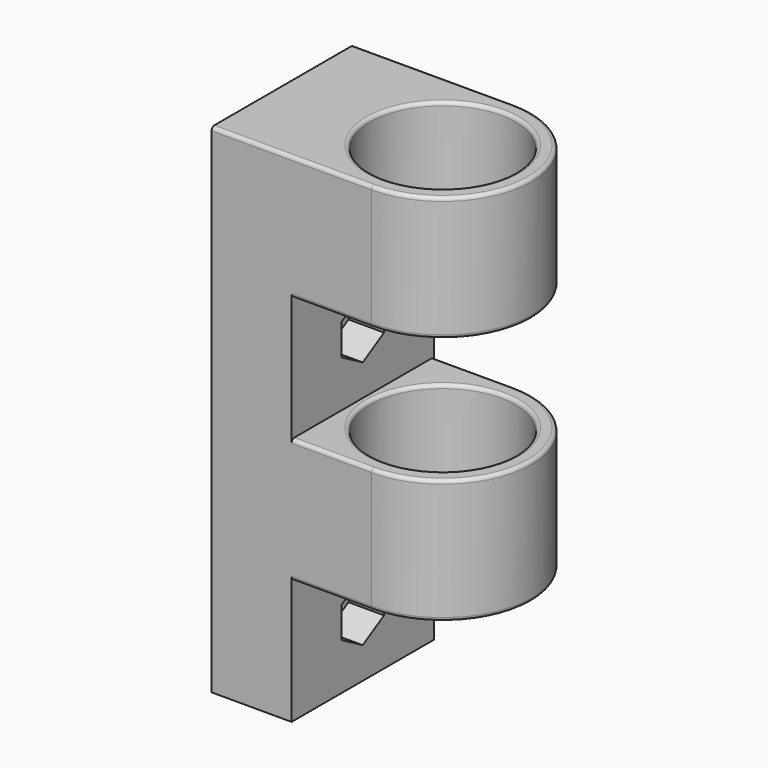
from build123d import *

# Parameters (mm, degrees)
F0_R     = 10.25
F1_DEPTH = 70
F2_W     = 11.25
F2_H     = 17.5
F2_W_2   = 18.7990599871
F3_DEPTH = 30
F4_R     = 2.1
F5_DEPTH = 5
F6_DEPTH = 11.251
F7_R     = 2.1
F8_DEPTH = 5
F9_DEPTH = 11.251
F10_R    = 0.5


# Not quite as in the source:
# - a feature names something its author has since deleted; it is built from what else it names


with BuildPart() as f1:
    # F0 (on Top) → F1 (new body)
    with BuildSketch(Plane.XY):
        with BuildLine():
            Line((0, 25), (0, 0))
            Line((0, 0), (22.5, 0))
            ThreePointArc((22.5, 0), (35, 12.5), (22.5, 25))
            Line((22.5, 25), (0, 25))
        make_face()
        with Locations((22.5, 12.5)):
            Circle(F0_R, mode=Mode.SUBTRACT)
    extrude(amount=F1_DEPTH)

    # F2 (on face) → F3 (cut)
    with BuildSketch(Plane.XZ):
        with Locations((16.875, 8.75)):
            Rectangle(F2_W, F2_H)
        with Locations((31.8995299935, 8.75)):
            Rectangle(F2_W_2, F2_H)
        with Locations((16.875, 43.75)):
            Rectangle(F2_W, F2_H)
        with Locations((31.8995299935, 43.75)):
            Rectangle(F2_W_2, F2_H)
    extrude(amount=-F3_DEPTH, mode=Mode.SUBTRACT)

    # F4 (on face) → F5 (cut)
    with BuildSketch(Plane.YZ.offset(11.25)):
        Polygon((16.25, 41.5849364905), (16.25, 45.9150635095), (12.5, 48.0801270189), (8.75, 45.9150635095), (8.75, 41.5849364905), (12.5, 39.4198729811), align=None)
        with Locations((12.5, 43.75)):
            Circle(F4_R, mode=Mode.SUBTRACT)
    extrude(amount=-F5_DEPTH, mode=Mode.SUBTRACT)

    # F6 (cut, through all): a face of the model
    f6_faces = [f1.faces().sort_by_distance(p)[0] for p in [
        (11.25, 12.5, 43.75),
    ]]
    extrude(f6_faces, amount=-F6_DEPTH, mode=Mode.SUBTRACT)

    # F7 (on face) → F8 (cut)
    with BuildSketch(Plane.YZ.offset(11.25)):
        Polygon((16.25, 6.5849364905), (16.25, 10.9150635095), (12.5, 13.0801270189), (8.75, 10.9150635095), (8.75, 6.5849364905), (12.5, 4.4198729811), align=None)
        with Locations((12.5, 8.75)):
            Circle(F7_R, mode=Mode.SUBTRACT)
    extrude(amount=-F8_DEPTH, mode=Mode.SUBTRACT)

    # F9 (cut, through all): a face of the model
    f9_faces = [f1.faces().sort_by_distance(p)[0] for p in [
        (11.25, 12.5, 8.75),
    ]]
    extrude(f9_faces, amount=-F9_DEPTH, mode=Mode.SUBTRACT)

    # F10
    f10_edges = [f1.edges().sort_by_distance(p)[0] for p in [
        (16.875, 0, 52.5),
        (16.875, 0, 35),
        (16.875, 0, 17.5),
        (12.25, 12.5, 17.5),
        (12.25, 12.5, 35),
        (12.25, 12.5, 52.5),
        (12.25, 12.5, 70),
        (35, 12.5, 70),
    ]]
    fillet(f10_edges, radius=F10_R)


solid = f1.part
